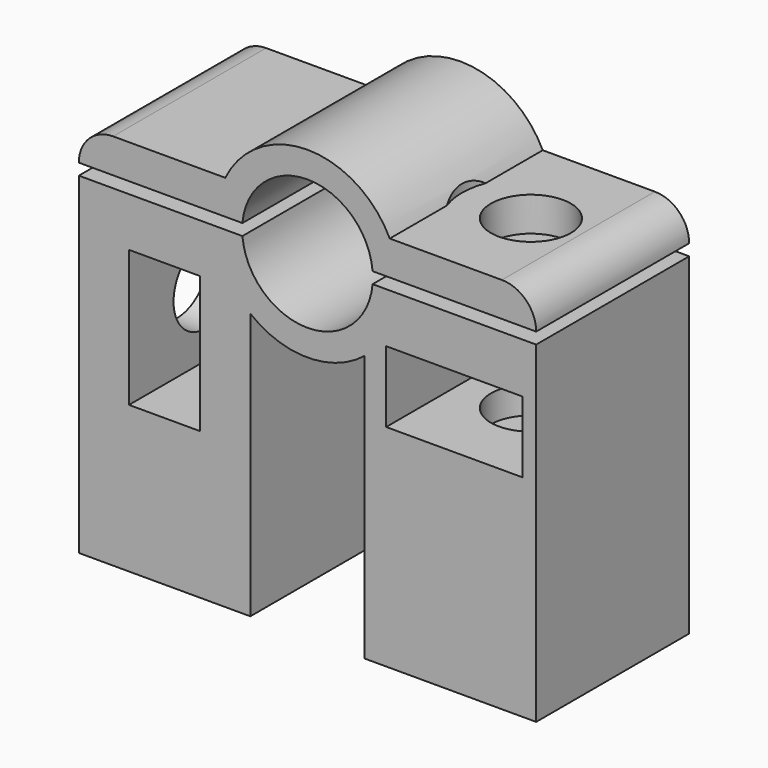
from build123d import *

# Parameters (mm, degrees)
F1_DEPTH  = 16.7254
F2_W      = 12.954
F2_H      = 27.051
F3_DEPTH  = 1.905
F4_R      = 3.4925
F5_DEPTH  = 10.668
F6_R      = 2.99999
F7_R      = 3.4925
F8_DEPTH  = 33.052
F9_R      = 3.4925
F10_DEPTH = 13
F11_W     = 6.223
F11_H     = 11.938
F11_W_2   = 11.938
F11_H_2   = 6.223
F12_DEPTH = 14.0775
F13_R     = 6.0325
F14_DEPTH = 25


# Not quite as in the source:
# - a fillet or chamfer is up to 0.001 mm smaller than in the source, because OpenCascade refuses the exact size
# - a length typed as a fraction of an inch, garbled in the dataset ("3 / 203.2 mm" for 3/8 in), is restored


with BuildPart() as f1:
    # F0 (on Front) → F1 (new body)
    with BuildSketch(Plane.XZ):
        with BuildLine():
            Line((-15, 0), (0, 0))
            Line((0, 0), (0, 29.051))
            Line((0, 29.051), (-14.3069142813, 29.051))
            ThreePointArc((-14.3069142813, 29.051), (-20, 23.836), (-25.6930857187, 29.051))
            Line((-25.6930857187, 29.051), (-40, 29.051))
            Line((-40, 29.051), (-40, 0))
            Line((-40, 0), (-25, 0))
            Line((-25, 0), (-25, 23.3060020016))
            ThreePointArc((-25, 23.3060020016), (-20, 21.551), (-15, 23.3060020016))
            Line((-15, 23.3060020016), (-15, 0))
        make_face()
    extrude(amount=F1_DEPTH)

    # F2 (on face) → F3 (cut)
    with BuildSketch(Plane(origin=(-40, 0, 0), x_dir=(0, -1, 0), z_dir=(-1, 0, 0))):
        with Locations((8.3627, 13.5255)):
            Rectangle(F2_W, F2_H)
    extrude(amount=-F3_DEPTH, mode=Mode.SUBTRACT)

    # F4 (on face) → F5 (cut)
    with BuildSketch(Plane(origin=(-38.095, 0, 0), x_dir=(0, -1, 0), z_dir=(-1, 0, 0))):
        with Locations((8.3627, 18.796)):
            Circle(F4_R)
    extrude(amount=-F5_DEPTH, mode=Mode.SUBTRACT)

    # F9 (on face) → F10 (cut)
    with BuildSketch(Plane.XY.offset(29.051)):
        with Locations((-7.1534571407, -8.3629)):
            Circle(F9_R)
    extrude(amount=-F10_DEPTH, mode=Mode.SUBTRACT)

    # F11 (on face) → F12 (cut)
    with BuildSketch(Plane.XZ.offset(16.7254)):
        with Locations((-32.5, 18.796)):
            Rectangle(F11_W, F11_H)
        with Locations((-7.1534571407, 21.551)):
            Rectangle(F11_W_2, F11_H_2)
    extrude(amount=-F12_DEPTH, mode=Mode.SUBTRACT)


with BuildPart() as f1b:
    # F0 (on Front) → F1, piece 2 (new body)
    with BuildSketch(Plane.XZ):
        with BuildLine():
            ThreePointArc((-25.6930857187, 30.051), (-20, 35.266), (-14.3069142813, 30.051))
            Line((-14.3069142813, 30.051), (0, 30.051))
            Line((0, 30.051), (0, 33.051))
            Line((0, 33.051), (-12.806252715, 33.051))
            ThreePointArc((-12.806252715, 33.051), (-20, 37.551), (-27.193747285, 33.051))
            Line((-27.193747285, 33.051), (-40, 33.051))
            Line((-40, 33.051), (-40, 30.051))
            Line((-40, 30.051), (-25.6930857187, 30.051))
        make_face()
    extrude(amount=F1_DEPTH)

    # F6 (radius 3 in the source; OpenCascade refuses exactly that, so slightly less here)
    f6_edges = [f1b.edges().sort_by_distance(p)[0] for p in [
        (-40, -8.3627, 33.051),
        (0, -8.3627, 33.051),
    ]]
    fillet(f6_edges, radius=F6_R)

    # F7 (on face) → F8 (cut, through all)
    with BuildSketch(Plane.XY.offset(33.051)):
        with Locations((-7.1534571407, -8.3629)):
            Circle(F7_R)
    extrude(amount=-F8_DEPTH, mode=Mode.SUBTRACT)

    # F13 (on face) → F14 (cut)
    with BuildSketch(Plane.XY.offset(33.051)):
        with Locations((-7.1534571407, -8.3629)):
            Circle(F13_R)
    extrude(amount=F14_DEPTH, mode=Mode.SUBTRACT)


solid = Compound([f1.part, f1b.part])
